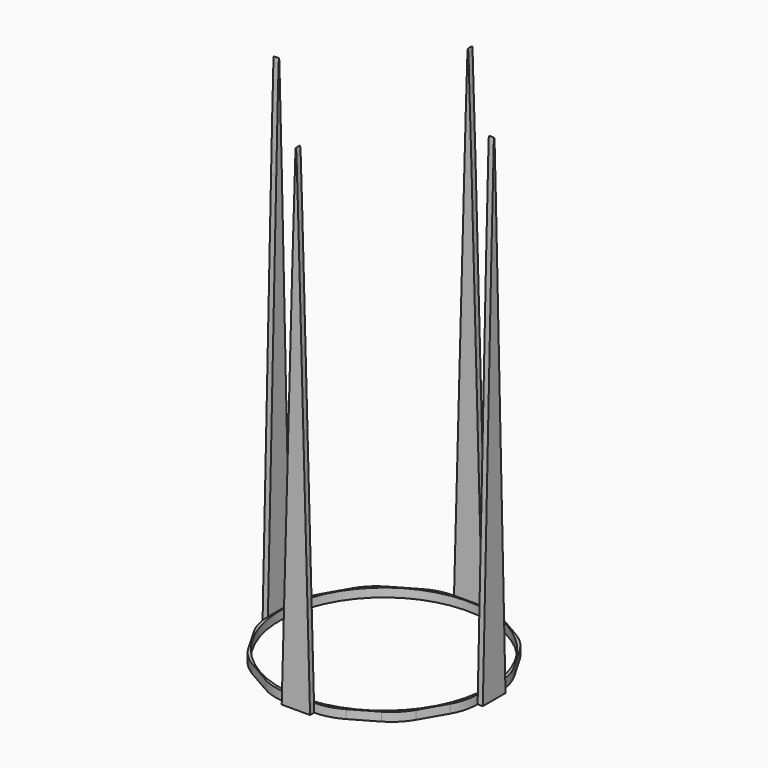
from build123d import *

# Parameters (mm, degrees)
F0_R        = 152.4
F1_DEPTH    = 12.7
F2_R        = 76.2
F4_DEPTH    = 7.62
F5_T1_DEPTH = 939.6748590095
F7_COUNT    = 4
F7_ANGLE    = 270


# Not quite as in the source:
# - a fillet or chamfer that OpenCascade refuses, or shapes differently, is made with other operations: its cross-section is extruded or revolved along the edge and cut away or added
# - a feature of the source that left no trace in its solid (it failed there, or was rolled back) is left out


with BuildPart() as f1:
    # F0 (on Top) → F1 (new body)
    with BuildSketch(Plane.XY):
        Polygon((-153.67, -41.1757524009), (-112.4942475991, -112.4942475991), (-41.1757524009, -153.67), (41.1757524009, -153.67), (112.4942475991, -112.4942475991), (153.67, -41.1757524009), (153.67, 41.1757524009), (112.4942475991, 112.4942475991), (41.1757524009, 153.67), (-41.1757524009, 153.67), (-112.4942475991, 112.4942475991), (-153.67, 41.1757524009), align=None)
        Circle(F0_R, mode=Mode.SUBTRACT)
    extrude(amount=F1_DEPTH)

    # F2
    f2_edges = [f1.edges().sort_by_distance(p)[0] for p in [
        (-41.175752, -153.67, 6.35),
        (41.175752, -153.67, 6.35),
        (112.494248, -112.494248, 6.35),
        (153.67, -41.175752, 6.35),
        (153.67, 41.175752, 6.35),
        (112.494248, 112.494248, 6.35),
        (41.175752, 153.67, 6.35),
        (-41.175752, 153.67, 6.35),
        (-112.494248, 112.494248, 6.35),
        (-153.67, 41.175752, 6.35),
        (-153.67, -41.175752, 6.35),
        (-112.494248, -112.494248, 6.35),
    ]]
    fillet(f2_edges, radius=F2_R)


with BuildPart() as f4:
    # F3 (on face) → F4 (new body)
    with BuildSketch(Plane.YZ.offset(153.67)):
        Polygon((-20.4119284295, 12.7), (-20.7580239376, 0), (20.7580239376, 0), (20.4119284295, 12.7), align=None)
        Polygon((0, 761.7172076579), (-20.4119284295, 12.7), (20.4119284295, 12.7), align=None)
    extrude(amount=F4_DEPTH)

    # F5: fillet of radius 5.08 on 1 edges, made by hand

    # F5_s2 → F5_t1 (cut)
    with BuildSketch(Plane.YZ.offset(-312.3574295047)):
        with BuildLine():
            add(Edge.make_bspline(
                [(5.0781147177, 575.3754164273), (0, 761.7172076579), (-5.0781147177, 575.3754164273)],
                knots=[0, 0, 0, 1, 1, 1], degree=2, weights=[1, 4, 1]))
            Line((-5.0781147177, 575.3754164273), (0, 761.7172076579))
            Line((0, 761.7172076579), (5.0781147177, 575.3754164273))
        make_face()
    extrude(amount=F5_T1_DEPTH, mode=Mode.SUBTRACT)


with BuildPart() as f7_1:
    # F7: instance of F4
    add(f4.part.rotate(Axis((0, 0, 12.7), (0, 0, 1)), 1 * F7_ANGLE / (F7_COUNT - 1)))


with BuildPart() as f7_2:
    # F7: instance of F4
    add(f4.part.rotate(Axis((0, 0, 12.7), (0, 0, 1)), 2 * F7_ANGLE / (F7_COUNT - 1)))


with BuildPart() as f7_3:
    # F7: instance of F4
    add(f4.part.rotate(Axis((0, 0, 12.7), (0, 0, 1)), 3 * F7_ANGLE / (F7_COUNT - 1)))


solid = Compound([f1.part, f4.part, f7_1.part, f7_2.part, f7_3.part])
